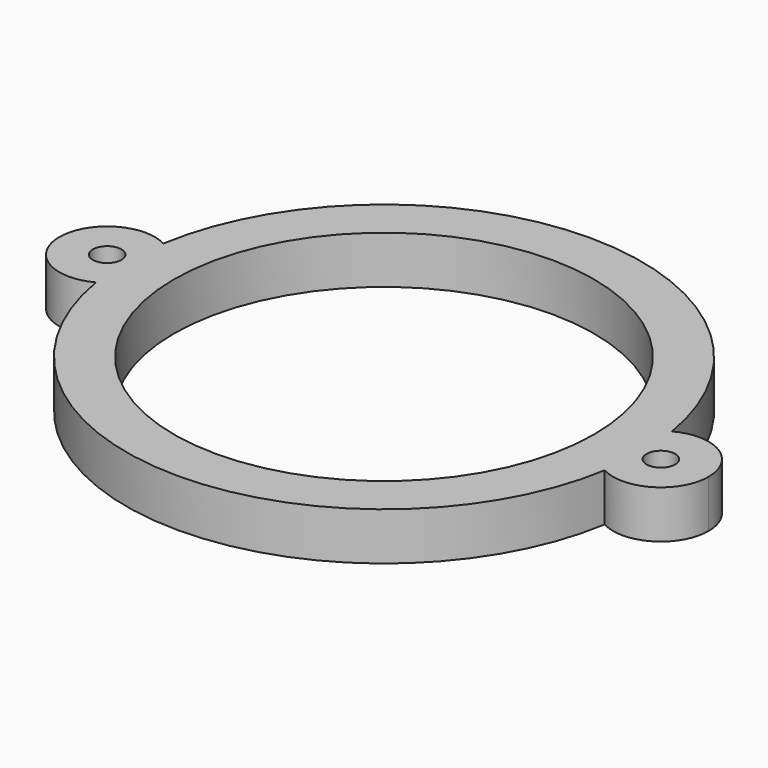
from build123d import *

# Parameters (mm, degrees)
F0_R     = 1.5
F1_DEPTH = 5
F2_DEPTH = 5
F3_R     = 22
F4_DEPTH = 6


with BuildPart() as f1:
    # F0 (on Top) → F1 (new body)
    with BuildSketch(Plane.XY):
        with BuildLine():
            ThreePointArc((-26.6379310345, -4.4068844099), (-27, 0), (-26.6379310345, 4.4068844099))
            ThreePointArc((-26.6379310345, 4.4068844099), (-34, 0), (-26.6379310345, -4.4068844099))
        make_face()
        with Locations((-29, 0)):
            Circle(F0_R, mode=Mode.SUBTRACT)
    extrude(amount=F1_DEPTH)



with BuildPart() as f1b:
    # F0 (on Top) → F1, piece 2 (new body)
    with BuildSketch(Plane.XY):
        with BuildLine():
            ThreePointArc((26.6379310345, 4.4068844099), (26.9093305187, 2.21086658), (27, 0))
            ThreePointArc((27, 0), (26.9093305187, -2.21086658), (26.6379310345, -4.4068844099))
            ThreePointArc((26.6379310345, -4.4068844099), (31.5680396388, -4.2901249881), (34, 0))
            ThreePointArc((34, 0), (31.5680396388, 4.2901249881), (26.6379310345, 4.4068844099))
        make_face()
        with Locations((29, 0)):
            Circle(F0_R, mode=Mode.SUBTRACT)
    extrude(amount=F1_DEPTH)


with BuildPart() as f1_1:
    add(f1.part)

    add(f1b.part)  # F2 merges F1b
    # F0 (on Top) → F2 (join)
    with BuildSketch(Plane.XY):
        with BuildLine():
            ThreePointArc((-24, 0), (-24.7098750119, 2.5680396388), (-26.6379310345, 4.4068844099))
            ThreePointArc((-26.6379310345, 4.4068844099), (-27, 0), (-26.6379310345, -4.4068844099))
            ThreePointArc((-26.6379310345, -4.4068844099), (-24.7098750119, -2.5680396388), (-24, 0))
        make_face()
        with BuildLine():
            ThreePointArc((26.6379310345, -4.4068844099), (26.9093305187, -2.21086658), (27, 0))
            ThreePointArc((27, 0), (26.9093305187, 2.21086658), (26.6379310345, 4.4068844099))
            ThreePointArc((26.6379310345, 4.4068844099), (24, 0), (26.6379310345, -4.4068844099))
        make_face()
        with BuildLine():
            ThreePointArc((26.6379310345, -4.4068844099), (24, 0), (26.6379310345, 4.4068844099))
            ThreePointArc((26.6379310345, 4.4068844099), (0, 27), (-26.6379310345, 4.4068844099))
            ThreePointArc((-26.6379310345, 4.4068844099), (-24.7098750119, 2.5680396388), (-24, 0))
            ThreePointArc((-24, 0), (-24.7098750119, -2.5680396388), (-26.6379310345, -4.4068844099))
            ThreePointArc((-26.6379310345, -4.4068844099), (0, -27), (26.6379310345, -4.4068844099))
        make_face()
    extrude(amount=F2_DEPTH)

    # F3 (on face) → F4 (cut)
    with BuildSketch(Plane.XY.offset(5)):
        Circle(F3_R)
    extrude(amount=-F4_DEPTH, mode=Mode.SUBTRACT)


solid = f1_1.part
